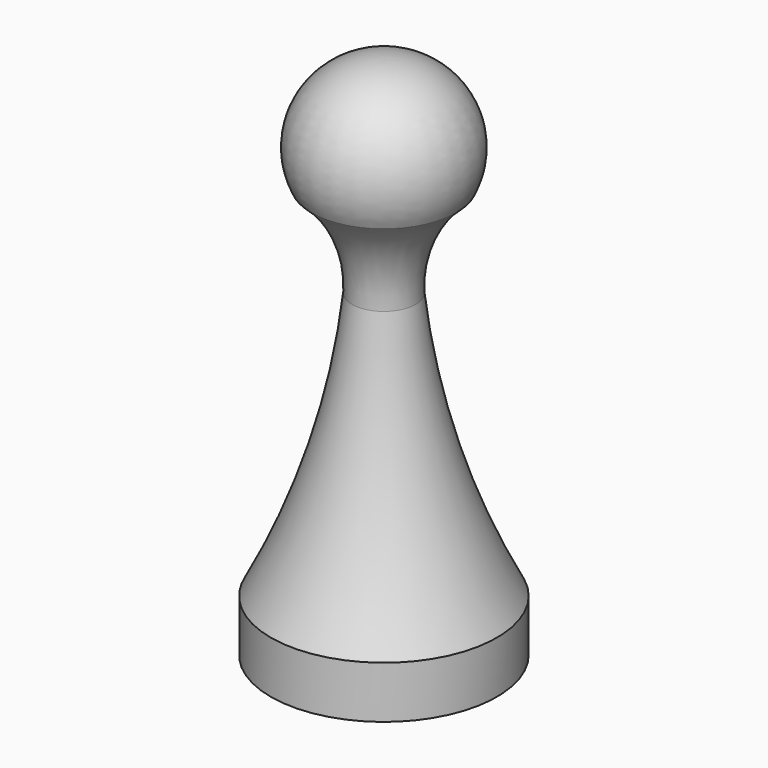
from build123d import *


# Not quite as in the source:
# - a feature of the source that left no trace in its solid (it failed there, or was rolled back) is left out


with BuildPart() as f1:
    # F0 (on Front) → F1 (revolve)
    with BuildSketch(Plane.XZ):
        with BuildLine():
            Line((0, 0), (0, 59.4318918884))
            ThreePointArc((0, 59.4318918884), (-7.6825377996, 55.4198742906), (-8.2024643198, 46.768438071))
            ThreePointArc((-8.2024643198, 46.768438071), (-4.6430967507, 41.9875630921), (-3.597572213, 36.1196212471))
            ThreePointArc((-3.597572213, 36.1196212471), (-6.7547874228, 20.5686230303), (-12.8073552623, 5.9000179172))
            Line((-12.8073552623, 5.9000179172), (-12.8073552623, 0))
            Line((-12.8073552623, 0), (0, 0))
        make_face()
    revolve(axis=Axis((0, 0, 29.7159459442), (0, 0, -1)))


solid = f1.part
